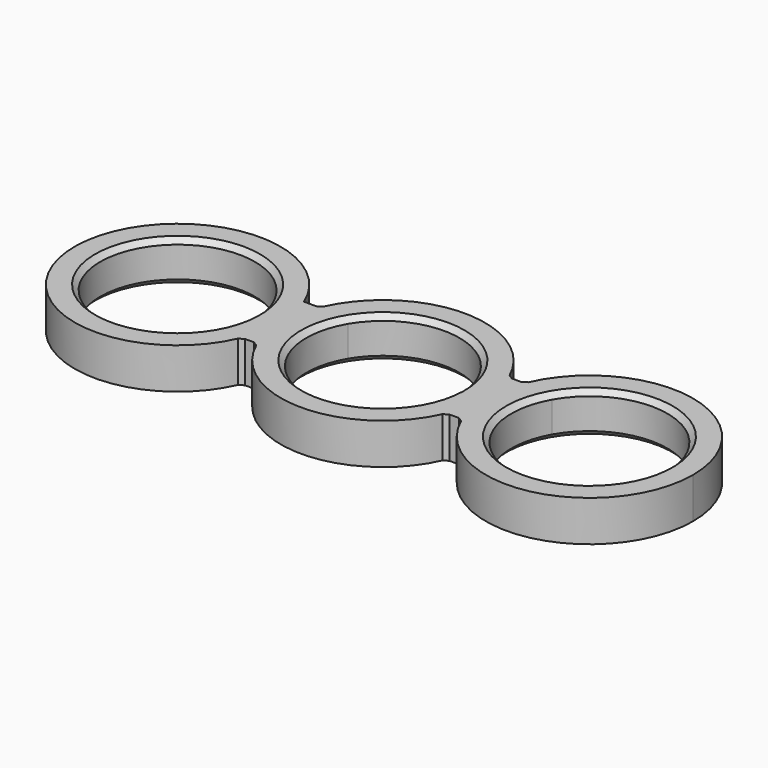
from build123d import *

# Parameters (mm, degrees)
F1_DEPTH    = 8
F2_T1_DEPTH = 8


# Not quite as in the source:
# - a fillet or chamfer that OpenCascade refuses, or shapes differently, is made with other operations: its cross-section is extruded or revolved along the edge and cut away or added


with BuildPart() as f1:
    # F0 (on Top) → F1 (new body)
    with BuildSketch(Plane.XY):
        with BuildLine():
            ThreePointArc((12.9113873807, 7.6351866975), (14.4684278813, 3.9578522768), (15, 0))
            ThreePointArc((15, 0), (14.4684278813, -3.9578522768), (12.9113873807, -7.6351866975))
            Line((12.9113873807, -7.6351866975), (18.4852353, -7.6351866975))
            ThreePointArc((18.4852353, -7.6351866975), (19.6176541156, -3.8919978161), (20, 0))
            ThreePointArc((20, 0), (19.6176541156, 3.8919978161), (18.4852353, 7.6351866975))
            Line((18.4852353, 7.6351866975), (12.9113873807, 7.6351866975))
        make_face()
        with BuildLine():
            ThreePointArc((-12.9113873807, 7.6351866975), (0, 15), (12.9113873807, 7.6351866975))
            Line((12.9113873807, 7.6351866975), (18.4852353, 7.6351866975))
            ThreePointArc((18.4852353, 7.6351866975), (0, 20), (-18.4852353, 7.6351866975))
            Line((-18.4852353, 7.6351866975), (-12.9113873807, 7.6351866975))
        make_face()
        with BuildLine():
            Line((18.4852353, -7.6351866975), (12.9113873807, -7.6351866975))
            ThreePointArc((12.9113873807, -7.6351866975), (0, -15), (-12.9113873807, -7.6351866975))
            Line((-12.9113873807, -7.6351866975), (-18.4852353, -7.6351866975))
            ThreePointArc((-18.4852353, -7.6351866975), (0, -20), (18.4852353, -7.6351866975))
        make_face()
        with BuildLine():
            ThreePointArc((-12.9113873807, -7.6351866975), (-15, 0), (-12.9113873807, 7.6351866975))
            Line((-12.9113873807, 7.6351866975), (-18.4852353, 7.6351866975))
            ThreePointArc((-18.4852353, 7.6351866975), (-20, 0), (-18.4852353, -7.6351866975))
            Line((-18.4852353, -7.6351866975), (-12.9113873807, -7.6351866975))
        make_face()
        with BuildLine():
            Line((21.6526307541, 7.6351866975), (18.4852353, 7.6351866975))
            ThreePointArc((18.4852353, 7.6351866975), (19.6176541156, 3.8919978161), (20, 0))
            ThreePointArc((20, 0), (19.6176541156, -3.8919978161), (18.4852353, -7.6351866975))
            Line((18.4852353, -7.6351866975), (21.6526307541, -7.6351866975))
            ThreePointArc((21.6526307541, -7.6351866975), (20.1620412737, 0), (21.6526307541, 7.6351866975))
        make_face()
        with BuildLine():
            ThreePointArc((-18.4852353, -7.6351866975), (-20, 0), (-18.4852353, 7.6351866975))
            Line((-18.4852353, 7.6351866975), (-21.5730507637, 7.6351866975))
            ThreePointArc((-21.5730507637, 7.6351866975), (-20.4496870957, 3.8908164426), (-20.0704748243, 0))
            ThreePointArc((-20.0704748243, 0), (-20.4496870957, -3.8908164426), (-21.5730507637, -7.6351866975))
            Line((-21.5730507637, -7.6351866975), (-18.4852353, -7.6351866975))
        make_face()
        with BuildLine():
            Line((27.135123316, 7.6351866975), (21.6526307541, 7.6351866975))
            ThreePointArc((21.6526307541, 7.6351866975), (20.1620412737, 0), (21.6526307541, -7.6351866975))
            Line((21.6526307541, -7.6351866975), (27.135123316, -7.6351866975))
            Line((27.135123316, -7.6351866975), (27.135123316, -7.5155344287))
            ThreePointArc((27.135123316, -7.5155344287), (25.1620412737, 0), (27.135123316, 7.5155344287))
            Line((27.135123316, 7.5155344287), (27.135123316, 7.6351866975))
        make_face()
        with BuildLine():
            ThreePointArc((60.7620412737, 0), (44.3517049129, 19.9238680174), (21.6526307541, 7.6351866975))
            Line((21.6526307541, 7.6351866975), (27.135123316, 7.6351866975))
            Line((27.135123316, 7.6351866975), (27.135123316, 7.5155344287))
            ThreePointArc((27.135123316, 7.5155344287), (44.347151005, 14.7985108162), (55.7620412737, 0))
            ThreePointArc((55.7620412737, 0), (44.347151005, -14.7985108162), (27.135123316, -7.5155344287))
            Line((27.135123316, -7.5155344287), (27.135123316, -7.6351866975))
            Line((27.135123316, -7.6351866975), (21.6526307541, -7.6351866975))
            ThreePointArc((21.6526307541, -7.6351866975), (44.3517049129, -19.9238680174), (60.7620412737, 0))
        make_face()
        with BuildLine():
            Line((-27.135123316, 7.6351866975), (-21.5730507637, 7.6351866975))
            ThreePointArc((-21.5730507637, 7.6351866975), (-60.3704748243, 0), (-21.5730507637, -7.6351866975))
            Line((-21.5730507637, -7.6351866975), (-27.135123316, -7.6351866975))
            ThreePointArc((-27.135123316, -7.6351866975), (-55.3704748243, 0), (-27.135123316, 7.6351866975))
        make_face()
        with BuildLine():
            ThreePointArc((-20.0704748243, 0), (-20.4496870957, 3.8908164426), (-21.5730507637, 7.6351866975))
            Line((-21.5730507637, 7.6351866975), (-27.135123316, 7.6351866975))
            ThreePointArc((-27.135123316, 7.6351866975), (-25.5957427695, 3.9547076156), (-25.0704748243, 0))
            ThreePointArc((-25.0704748243, 0), (-25.5957427695, -3.9547076156), (-27.135123316, -7.6351866975))
            Line((-27.135123316, -7.6351866975), (-21.5730507637, -7.6351866975))
            ThreePointArc((-21.5730507637, -7.6351866975), (-20.4496870957, -3.8908164426), (-20.0704748243, 0))
        make_face()
    extrude(amount=F1_DEPTH)

    # F2: chamfer of 1 on 13 edges, made by hand

    # F2_s2 → F2_t1 (join)
    with BuildSketch(Plane.XY):
        with BuildLine():
            Line((20.9909460118, -7.6351866975), (21.9050819396, -8.2297788713))
            ThreePointArc((21.9050819396, -8.2297788713), (21.7829852925, -7.9487651651), (21.6526307541, -7.6351866975))
            Line((21.6526307541, -7.6351866975), (20.9909460118, -7.6351866975))
        make_face()
        with BuildLine():
            Line((-19.1424541452, -7.6351866975), (-18.2309087097, -8.2239873309))
            ThreePointArc((-18.2309087097, -8.2239873309), (-18.3538297184, -7.9458753243), (-18.4852353, -7.6351866975))
            Line((-18.4852353, -7.6351866975), (-19.1424541452, -7.6351866975))
        make_face()
        with BuildLine():
            Line((21.9050819396, 8.2297788713), (20.9909460118, 7.6351866975))
            Line((20.9909460118, 7.6351866975), (21.6526307541, 7.6351866975))
            ThreePointArc((21.6526307541, 7.6351866975), (21.7829852925, 7.9487651651), (21.9050819396, 8.2297788713))
        make_face()
        with BuildLine():
            Line((-18.2309087097, 8.2239873309), (-19.1424541452, 7.6351866975))
            Line((-19.1424541452, 7.6351866975), (-18.4852353, 7.6351866975))
            ThreePointArc((-18.4852353, 7.6351866975), (-18.3538297184, 7.9458753243), (-18.2309087097, 8.2239873309))
        make_face()
        with BuildLine():
            Line((19.1424541452, 7.6351866975), (18.2309087097, 8.2239873309))
            ThreePointArc((18.2309087097, 8.2239873309), (18.3538297184, 7.9458753243), (18.4852353, 7.6351866975))
            Line((18.4852353, 7.6351866975), (19.1424541452, 7.6351866975))
        make_face()
        with BuildLine():
            Line((19.1424541452, -7.6351866975), (18.2309087097, -8.2239873309))
            ThreePointArc((18.2309087097, -8.2239873309), (18.3538297184, -7.9458753243), (18.4852353, -7.6351866975))
            Line((18.4852353, -7.6351866975), (19.1424541452, -7.6351866975))
        make_face()
        with BuildLine():
            Line((-21.8264389289, -8.2269036385), (-20.9135835494, -7.6351866975))
            Line((-20.9135835494, -7.6351866975), (-21.5730507637, -7.6351866975))
            ThreePointArc((-21.5730507637, -7.6351866975), (-21.703929906, -7.9473306392), (-21.8264389289, -8.2269036385))
        make_face()
    extrude(amount=F2_T1_DEPTH)

    # F2_s3 → F2_t4 (revolve, cut)
    with BuildSketch(Plane(origin=(-10.2155381424, -17.5076147757, 0), x_dir=(0, 0, 1), z_dir=(0.5039727193, 0.8637195715, 0))):
        Polygon((8, -18.5892112809), (7, -19.5892112809), (8, -19.5892112809), align=None)
    revolve(axis=Axis((-40.2204748243, 0, 8), (0, 0, -1)), mode=Mode.SUBTRACT)

    # F2_s5 → F2_t6 (revolve, cut)
    with BuildSketch(Plane(origin=(0, 0, 0), x_dir=(0, 0, 1), z_dir=(0.5090124465, -0.8607591587, 0))):
        Polygon((7, 15), (8, 16), (8, 15), align=None)
    revolve(axis=Axis((0, 0, 8), (0, 0, -1)), mode=Mode.SUBTRACT)

    # F2_s7 → F2_t8 (revolve, cut)
    with BuildSketch(Plane(origin=(9.7630309126, 17.3122900606, 0), x_dir=(0, 0, 1), z_dir=(-0.4912114006, -0.8710403894, 0))):
        Polygon((8, -18.9440721866), (7, -19.9440721866), (8, -19.9440721866), align=None)
    revolve(axis=Axis((40.4620412737, 0, 8), (0, 0, -1)), mode=Mode.SUBTRACT)

    # F2_s9 → F2_t10 (revolve, cut)
    with BuildSketch(Plane(origin=(-10.2155381424, -17.5076147757, 0), x_dir=(0, 0, 1), z_dir=(0.5039727193, 0.8637195715, 0))):
        Polygon((0, -18.5892112809), (1, -19.5892112809), (0, -19.5892112809), align=None)
    revolve(axis=Axis((-40.2204748243, 0, 0), (0, 0, -1)), mode=Mode.SUBTRACT)

    # F2_s11 → F2_t12 (revolve, cut)
    with BuildSketch(Plane(origin=(0, 0, 0), x_dir=(0, 0, 1), z_dir=(0.5090124465, -0.8607591587, 0))):
        Polygon((1, 15), (0, 16), (0, 15), align=None)
    revolve(axis=Axis((0, 0, 0), (0, 0, -1)), mode=Mode.SUBTRACT)

    # F2_s13 → F2_t14 (revolve, cut)
    with BuildSketch(Plane(origin=(9.7630309126, 17.3122900606, 0), x_dir=(0, 0, 1), z_dir=(-0.4912114006, -0.8710403894, 0))):
        Polygon((0, -18.9440721866), (1, -19.9440721866), (0, -19.9440721866), align=None)
    revolve(axis=Axis((40.4620412737, 0, 0), (0, 0, -1)), mode=Mode.SUBTRACT)


solid = f1.part
